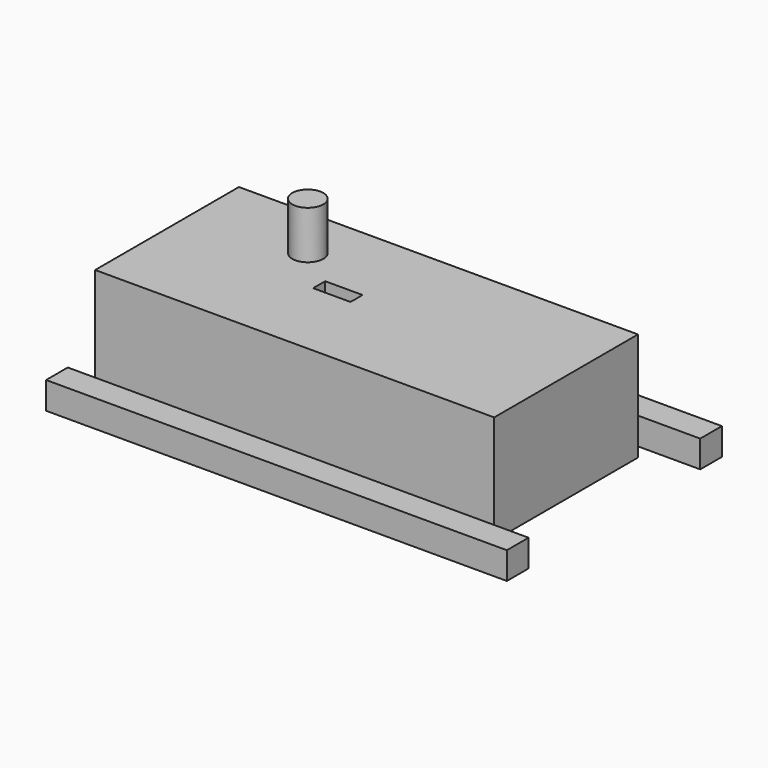
from build123d import *

# Parameters (mm, degrees)
F0_W         = 147.224877195
F0_H         = 66.3036294561
F0_R         = 5.7267932756
F1_DEPTH     = 10
F0_W_2       = 170
F0_H_2       = 10
F1_FACE_W    = 147.224877195
F1_FACE_H    = 66.3036294561
F1_FACE_W_2  = 65.479831006
F1_FACE_H_2  = 5.5599757362
F1_FACE_R    = 5.7267932756
F1_FACE1_W   = 147.224877195
F1_FACE1_H   = 66.3036294561
F1_FACE1_W_2 = 65.479831006
F1_FACE1_H_2 = 5.5599757362
F1_FACE1_R   = 5.7267932756
F2_DEPTH     = 30
F3_DEPTH     = 25
F4_DEPTH     = 47.7


# Not quite as in the source:
# - the program builds the solid bodies; features that only make, move or delete a surface that nothing else refers to are left out


with BuildPart() as f1:
    # F0 (on Top) → F1 (new body)
    with BuildSketch(Plane.XY):
        with Locations((-8.8865962121, 0)):
            Rectangle(F0_W, F0_H)
        with BuildLine():
            ThreePointArc((-12.689527612, -2.7799878681), (-69.902287741, 0), (-12.689527612, 2.7799878681))
            Line((-12.689527612, 2.7799878681), (39.1101999373, 2.7799878681))
            Line((39.1101999373, 2.7799878681), (39.1101999373, -2.7799878681))
            Line((39.1101999373, -2.7799878681), (-12.689527612, -2.7799878681))
        make_face(mode=Mode.SUBTRACT)
        with BuildLine():
            Line((-26.3696310687, 2.7799878681), (-12.689527612, 2.7799878681))
            ThreePointArc((-12.689527612, 2.7799878681), (-69.902287741, 0), (-12.689527612, -2.7799878681))
            Line((-12.689527612, -2.7799878681), (-26.3696310687, -2.7799878681))
            Line((-26.3696310687, -2.7799878681), (-26.3696310687, 2.7799878681))
        make_face()
        with Locations((-41.2283673889, 13.3251665685)):
            Circle(F0_R, mode=Mode.SUBTRACT)
    extrude(amount=-F1_DEPTH)

    # F0 (on Top) + F1_face (on face) + F1_face1 (on face) → F2 (join)
    with BuildSketch(Plane.XY):
        with BuildLine():
            Line((-26.3696310687, 2.7799878681), (-12.689527612, 2.7799878681))
            ThreePointArc((-12.689527612, 2.7799878681), (-69.902287741, 0), (-12.689527612, -2.7799878681))
            Line((-12.689527612, -2.7799878681), (-26.3696310687, -2.7799878681))
            Line((-26.3696310687, -2.7799878681), (-26.3696310687, 2.7799878681))
        make_face()
        with Locations((-41.2283673889, 13.3251665685)):
            Circle(F0_R, mode=Mode.SUBTRACT)
        with BuildLine():
            ThreePointArc((-12.689527612, 2.7799878681), (-12.5882370901, 1.3916338697), (-12.5544470368, 0))
            ThreePointArc((-12.5544470368, 0), (-12.5882370901, -1.3916338697), (-12.689527612, -2.7799878681))
            Line((-12.689527612, -2.7799878681), (39.1101999373, -2.7799878681))
            Line((39.1101999373, -2.7799878681), (39.1101999373, 2.7799878681))
            Line((39.1101999373, 2.7799878681), (-12.689527612, 2.7799878681))
        make_face()
    with BuildSketch(Plane(origin=(-9.1256930522, -0.1477141359, 0), x_dir=(1, 0, 0), z_dir=(0, 0, 1))):
        with Locations((0.2390968402, 0.1477141359)):
            Rectangle(F1_FACE_W, F1_FACE_H)
        with Locations((15.4959774865, 0.1477141359)):
            Rectangle(F1_FACE_W_2, F1_FACE_H_2, mode=Mode.SUBTRACT)
        with Locations((-32.1026743367, 13.4728807044)):
            Circle(F1_FACE_R, mode=Mode.SUBTRACT)
    with BuildSketch(Plane(origin=(-9.1256930522, -0.1477141359, -10), x_dir=(1, 0, 0), z_dir=(0, 0, -1))):
        with Locations((0.2390968402, -0.1477141359)):
            Rectangle(F1_FACE1_W, F1_FACE1_H)
        with Locations((15.4959774865, -0.1477141359)):
            Rectangle(F1_FACE1_W_2, F1_FACE1_H_2, mode=Mode.SUBTRACT)
        with Locations((-32.1026743367, -13.4728807044)):
            Circle(F1_FACE1_R, mode=Mode.SUBTRACT)
    extrude(amount=F2_DEPTH, dir=(0, 0, 1))

    # F0 (on Top) → F4 (join)
    with BuildSketch(Plane.XY):
        with Locations((-41.2283673889, 13.3251665685)):
            Circle(F0_R)
    extrude(amount=F4_DEPTH)


with BuildPart() as f1b:
    # F0 (on Top) → F1, piece 2 (new body)
    with BuildSketch(Plane.XY):
        with Locations((-1.6613137935, -45.5752154062)):
            Rectangle(F0_W_2, F0_H_2)
    extrude(amount=-F1_DEPTH)


with BuildPart() as f1c:
    # F0 (on Top) → F1, piece 3 (new body)
    with BuildSketch(Plane.XY):
        with Locations((-1.6613137935, 43.5946881741)):
            Rectangle(F0_W_2, F0_H_2)
    extrude(amount=-F1_DEPTH)


with BuildPart() as f3:
    # F0 (on Top) → F3 (new body)
    with BuildSketch(Plane.XY):
        with BuildLine():
            ThreePointArc((-12.689527612, -2.7799878681), (-12.5882370901, -1.3916338697), (-12.5544470368, 0))
            ThreePointArc((-12.5544470368, 0), (-12.5882370901, 1.3916338697), (-12.689527612, 2.7799878681))
            Line((-12.689527612, 2.7799878681), (-26.3696310687, 2.7799878681))
            Line((-26.3696310687, 2.7799878681), (-26.3696310687, -2.7799878681))
            Line((-26.3696310687, -2.7799878681), (-12.689527612, -2.7799878681))
        make_face()
    extrude(amount=F3_DEPTH)


solid = Compound([f1.part, f1b.part, f1c.part, f3.part])
